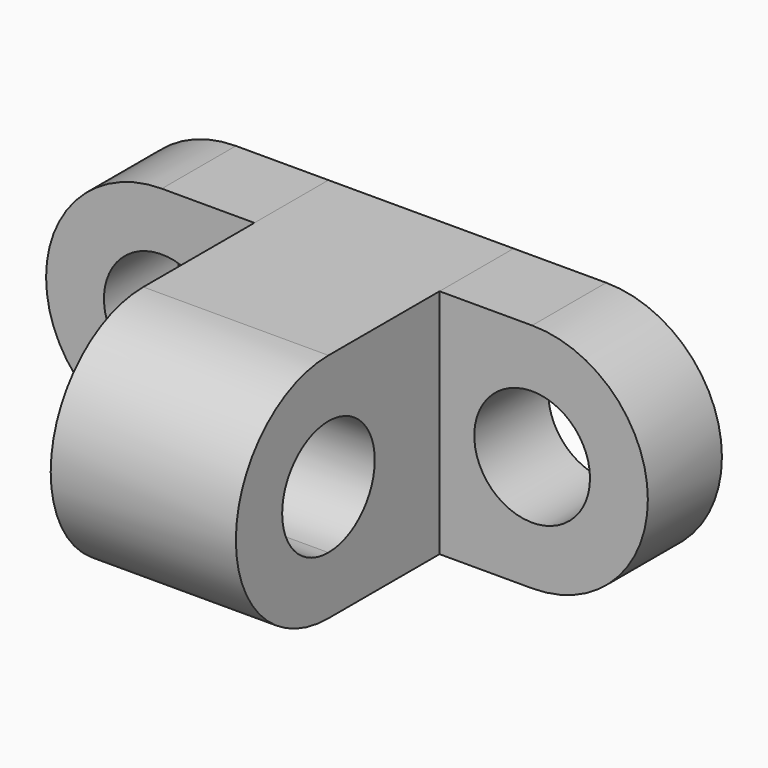
from build123d import *
from build123d import SkipClean  # not in build123d's __all__

# Parameters (mm, degrees)
F0_R     = 12.5
F1_DEPTH = 20
F0_W     = 40
F0_H     = 50
F2_DEPTH = 50
F4_DEPTH = 40
F5_DEPTH = 85.001


with BuildPart() as f1:
    # F0 (on Front) → F1 (new body)
    with BuildSketch(Plane.XZ):
        with BuildLine():
            Line((20, 50), (0, 50))
            ThreePointArc((0, 50), (-25, 25), (0, 0))
            Line((0, 0), (20, 0))
            Line((20, 0), (20, 50))
        make_face()
        with Locations((0, 25)):
            Circle(F0_R, mode=Mode.SUBTRACT)
    extrude(amount=F1_DEPTH)


with BuildPart() as f1b:
    # F0 (on Front) → F1, piece 2 (new body)
    with BuildSketch(Plane.XZ):
        with BuildLine():
            Line((80, 50), (60, 50))
            Line((60, 50), (60, 0))
            Line((60, 0), (80, 0))
            ThreePointArc((80, 0), (105, 25), (80, 50))
        make_face()
        with Locations((80, 25)):
            Circle(F0_R, mode=Mode.SUBTRACT)
    extrude(amount=F1_DEPTH)


with BuildPart() as f2:
    # F0 (on Front) → F2 (new body)
    with BuildSketch(Plane.XZ):
        with Locations((40, 25)):
            Rectangle(F0_W, F0_H)
    extrude(amount=F2_DEPTH)

    # F3 (on face) → F4 (join, through all)
    with BuildSketch(Plane(origin=(20, 0, 0), x_dir=(0, -1, 0), z_dir=(-1, 0, 0))):
        with BuildLine():
            ThreePointArc((50, 37.5), (37.5, 25), (50, 12.5))
            Line((50, 12.5), (50, 37.5))
        make_face()
        with BuildLine():
            Line((50, 12.5), (50, 0))
            ThreePointArc((50, 0), (75, 25), (50, 50))
            Line((50, 50), (50, 37.5))
            ThreePointArc((50, 37.5), (58.8388347648, 33.8388347648), (62.5, 25))
            ThreePointArc((62.5, 25), (58.8388347648, 16.1611652352), (50, 12.5))
        make_face()
    extrude(amount=-F4_DEPTH)

    # F3 (on face) → F5 (cut, through all)
    with BuildSketch(Plane(origin=(20, 0, 0), x_dir=(0, -1, 0), z_dir=(-1, 0, 0))):
        with BuildLine():
            ThreePointArc((50, 37.5), (37.5, 25), (50, 12.5))
            Line((50, 12.5), (50, 37.5))
        make_face()
    with SkipClean():  # cleaning this boolean's faces spoils the solid; the shape is the same uncleaned
        extrude(amount=-F5_DEPTH, mode=Mode.SUBTRACT)


solid = Compound([f1.part, f1b.part, f2.part])
